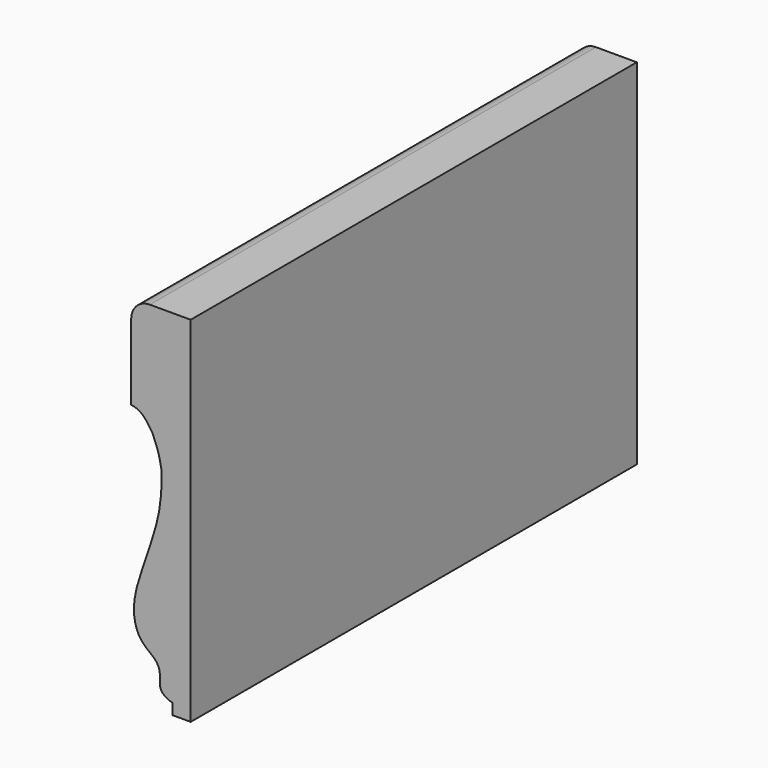
from build123d import *

# Parameters (mm, degrees)
F1_DEPTH = 150
F2_R     = 5


with BuildPart() as f1:
    # F0 (on Front) → F1 (new body)
    with BuildSketch(Plane.XZ):
        with BuildLine():
            Line((34.1070947651, -11.6565211154), (34.1070947651, 83.5819763541))
            Line((34.1070947651, 83.5819763541), (18.1070947651, 83.5819763541))
            Line((18.1070947651, 83.5819763541), (18.1070947651, 58.2385096952))
            add(Edge.make_bspline(
                [(18.1070947651, 58.2385096952), (18.9126885015, 58.0648723833), (20.9066399185, 57.6533927421), (22.9699261319, 54.8647603074), (23.8345864999, 53.365067498)],
                knots=[0, 0, 0, 0, 0.4194906876, 1, 1, 1, 1], degree=3))
            add(Edge.make_bspline(
                [(23.8345864999, 53.365067498), (25.184784915, 50.2428744032), (25.5859287593, 49.2007282356), (26.16743222, 45.8712734469)],
                knots=[0, 0, 0, 0, 7.8485105869, 7.8485105869, 7.8485105869, 7.8485105869], degree=3))
            add(Edge.make_bspline(
                [(26.16743222, 45.8712734469), (26.398906107, 44.8603835421), (26.2909467908, 39.1556882934), (25.1251682729, 32.0158799134), (21.2520767217, 20.9130118261), (18.0035620712, 11.0653072942), (19.8976758362, 3.0803796745), (24.7880165178, 0.3532833446), (26.1726626976, -2.8377032419), (25.2579878267, -7.0729338973), (28.1889608146, -8.5198188357), (29.1828027494, -8.6572972648)],
                knots=[0, 0, 0, 0, 0.1089398672, 0.2331773817, 0.3848807802, 0.5289478889, 0.6496881605, 0.750125742, 0.8295349848, 0.9162766416, 1, 1, 1, 1], degree=3))
            Line((29.1828027494, -8.6572972648), (29.1828027494, -11.6565211154))
            Line((29.1828027494, -11.6565211154), (34.1070947651, -11.6565211154))
        make_face()
    extrude(amount=F1_DEPTH)

    # F2
    f2_edges = [f1.edges().sort_by_distance(p)[0] for p in [
        (18.107095, -75, 83.581976),
    ]]
    fillet(f2_edges, radius=F2_R)


solid = f1.part
